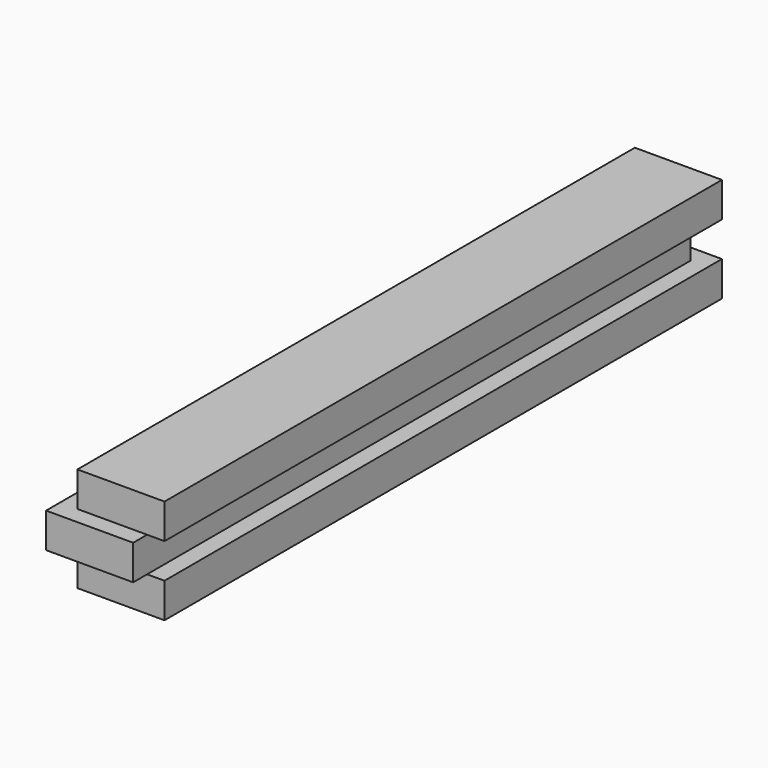
from build123d import *

# Parameters (mm, degrees)
F2_W     = 7.9375
F2_H     = 63.5
F3_DEPTH = 3.175
F4_W     = 7.9375
F4_H     = 63.5
F5_DEPTH = 3.175
F6_W     = 7.9375
F6_H     = 63.5
F7_DEPTH = 3.175


# Not quite as in the source:
# - a variable given as a bare number and used for a length is read in inches; the dataset says mm whatever the document's units were


with BuildPart() as f3:
    # F2 (on Top) → F3 (new body)
    with BuildSketch(Plane.XY):
        with Locations((3.96875, 31.75)):
            Rectangle(F2_W, F2_H)
    extrude(amount=F3_DEPTH)

    # F4 (on face) → F5 (join)
    with BuildSketch(Plane.XY.offset(3.175)):
        with Locations((2.38125, 30.1625)):
            Rectangle(F4_W, F4_H)
    extrude(amount=F5_DEPTH)

    # F6 (on face) → F7 (join)
    with BuildSketch(Plane.XY.offset(6.35)):
        with Locations((3.96875, 31.75)):
            Rectangle(F6_W, F6_H)
    extrude(amount=F7_DEPTH)


solid = f3.part
